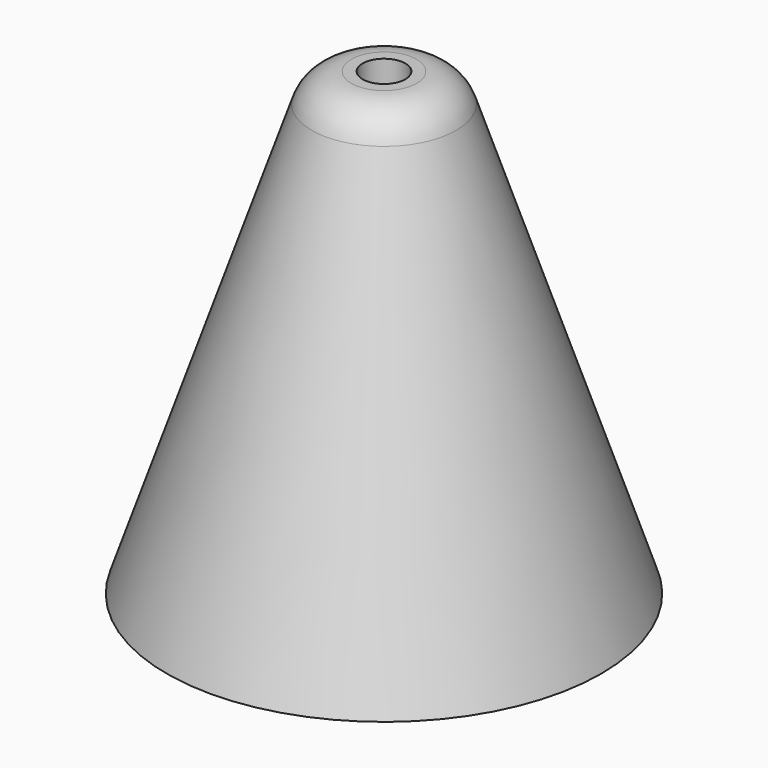
from build123d import *

# Parameters (mm, degrees)
F0_R      = 52
F4_R      = 15
F2_R      = 20
F6_R      = 50
F9_R      = 5.125
F10_DEPTH = 25
F11_R     = 10
F12_R     = 9.4


with BuildPart() as f5:
    # F0 (on Top) → F5 section 0
    with BuildSketch(Plane.XY):
        Circle(F0_R)
    # F4 (on offset) → F5 section 1
    with BuildSketch(Plane.XY.offset(110)):
        Circle(F4_R)
    loft()

    # F2 (on offset) → F7 section 0
    with BuildSketch(Plane.XY.offset(80)):
        Circle(F2_R)
    # F6 (on face) → F7 section 1
    with BuildSketch(Plane(origin=(0, 0, 0), x_dir=(1, 0, 0), z_dir=(0, 0, -1))):
        Circle(F6_R)
    loft(mode=Mode.SUBTRACT)

    # F9 (on face) → F10 (cut)
    with BuildSketch(Plane.XY.offset(110)):
        Circle(F9_R)
    extrude(amount=-F10_DEPTH, mode=Mode.SUBTRACT)

    # F11
    f11_edges = [f5.edges().sort_by_distance(p)[0] for p in [
        (-15, 0, 110),
    ]]
    fillet(f11_edges, radius=F11_R)

    # F12
    f12_edges = [f5.edges().sort_by_distance(p)[0] for p in [
        (-20, 0, 80),
    ]]
    fillet(f12_edges, radius=F12_R)


solid = f5.part
